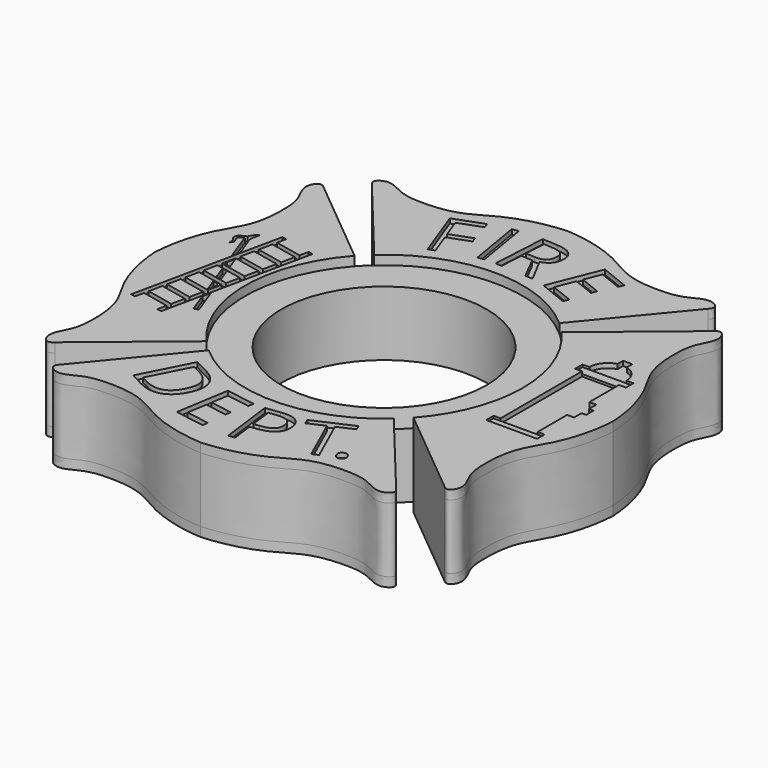
from build123d import *

# Parameters (mm, degrees)
F0_R            = 11.1
F1_DEPTH        = 7
F2_DEPTH        = 8
F3_DEPTH        = 1
F5_DEPTH        = 9.5
F6_DEPTH        = 0.5
F7_DEPTH        = 1
F9_DEPTH        = 9.5
F10_DEPTH       = 0.25
F11_DEPTH       = 0.5
F13_DEPTH       = 0.75
F14_DEPTH       = 1
F15_TEXT_SIZE   = 8.3333333333
F15_TEXT_SIZE_2 = 8.3471097203
F16_DEPTH       = 0.5
F17_TEXT_SIZE   = 8.3333333333
F17_TEXT_SIZE_2 = 8.125
F18_DEPTH       = 0.5


# Not quite as in the source:
# - Text() gives the source's letters only with a copy of the font that has no kerning and outlines rounded to 1/6400 em; it was checked with that copy


with BuildPart() as f1:
    # F0 (on Top) → F1 (new body)
    with BuildSketch(Plane.XY):
        with BuildLine():
            ThreePointArc((-11.1803398875, -10), (-15, 0), (-11.1803398875, 10))
            Line((-11.1803398875, 10), (-21.0544988513, 18.1538552022))
            add(Edge.make_bspline(
                [(-21.0544988513, 18.1538552022), (-21.4950011151, 18.5812700665), (-22.1300751643, 18.2333823026), (-22.4613402272, 16.9307561885), (-21.2849791288, 15.2167799257), (-21.0671926921, 12.725478547), (-21.3396788346, 9.0490697928), (-23.5217250696, 6.0536176188), (-24.5760919224, 2.2657519289), (-24.7081988852, 0.6627934752), (-24.7611551091, 0)],
                knots=[0, 0, 0, 0, 0.0790627116, 0.1662291191, 0.279613322, 0.4082260353, 0.5616601797, 0.7190317703, 0.8790842796, 1, 1, 1, 1], degree=3))
            add(Edge.make_bspline(
                [(-21.0544988513, -18.1538552022), (-21.4950011151, -18.5812700665), (-22.1300751643, -18.2333823026), (-22.4613402272, -16.9307561885), (-21.2849791288, -15.2167799257), (-21.0671926921, -12.725478547), (-21.3396788346, -9.0490697928), (-23.5217250696, -6.0536176188), (-24.5760919224, -2.2657519289), (-24.7081988852, -0.6627934752), (-24.7611551091, 0)],
                knots=[0, 0, 0, 0, 0.0790627116, 0.1662291191, 0.279613322, 0.4082260353, 0.5616601797, 0.7190317703, 0.8790842796, 1, 1, 1, 1], degree=3))
            Line((-21.0544988513, -18.1538552022), (-11.1803398875, -10))
        make_face()
        with BuildLine():
            ThreePointArc((-10, 11.1803398875), (0, 15), (10, 11.1803398875))
            Line((10, 11.1803398875), (18.1538552022, 21.0544988513))
            add(Edge.make_bspline(
                [(18.1538552022, 21.0544988513), (18.5812700665, 21.4950011151), (18.2333823026, 22.1300751643), (16.9307561885, 22.4613402272), (15.2167799257, 21.2849791288), (12.725478547, 21.0671926921), (9.0490697928, 21.3396788346), (6.0536176188, 23.5217250696), (2.2657519289, 24.5760919224), (0.6627934752, 24.7081988852), (0, 24.7611551091)],
                knots=[0, 0, 0, 0, 0.0790627116, 0.1662291191, 0.279613322, 0.4082260353, 0.5616601797, 0.7190317703, 0.8790842796, 1, 1, 1, 1], degree=3))
            add(Edge.make_bspline(
                [(-18.1538552022, 21.0544988513), (-18.5812700665, 21.4950011151), (-18.2333823026, 22.1300751643), (-16.9307561885, 22.4613402272), (-15.2167799257, 21.2849791288), (-12.725478547, 21.0671926921), (-9.0490697928, 21.3396788346), (-6.0536176188, 23.5217250696), (-2.2657519289, 24.5760919224), (-0.6627934752, 24.7081988852), (0, 24.7611551091)],
                knots=[0, 0, 0, 0, 0.0790627116, 0.1662291191, 0.279613322, 0.4082260353, 0.5616601797, 0.7190317703, 0.8790842796, 1, 1, 1, 1], degree=3))
            Line((-18.1538552022, 21.0544988513), (-10, 11.1803398875))
        make_face()
        with BuildLine():
            ThreePointArc((11.1803398875, 10), (14.0125853844, 5.3523313466), (15, 0))
            ThreePointArc((15, 0), (14.0125853844, -5.3523313466), (11.1803398875, -10))
            Line((11.1803398875, -10), (21.0544988513, -18.1538552022))
            add(Edge.make_bspline(
                [(21.0544988513, -18.1538552022), (21.4950011151, -18.5812700665), (22.1300751643, -18.2333823026), (22.4613402272, -16.9307561885), (21.2849791288, -15.2167799257), (21.0671926921, -12.725478547), (21.3396788346, -9.0490697928), (23.5217250696, -6.0536176188), (24.5760919224, -2.2657519289), (24.7081988852, -0.6627934752), (24.7611551091, 0)],
                knots=[0, 0, 0, 0, 0.0790627116, 0.1662291191, 0.279613322, 0.4082260353, 0.5616601797, 0.7190317703, 0.8790842796, 1, 1, 1, 1], degree=3))
            add(Edge.make_bspline(
                [(21.0544988513, 18.1538552022), (21.4950011151, 18.5812700665), (22.1300751643, 18.2333823026), (22.4613402272, 16.9307561885), (21.2849791288, 15.2167799257), (21.0671926921, 12.725478547), (21.3396788346, 9.0490697928), (23.5217250696, 6.0536176188), (24.5760919224, 2.2657519289), (24.7081988852, 0.6627934752), (24.7611551091, 0)],
                knots=[0, 0, 0, 0, 0.0790627116, 0.1662291191, 0.279613322, 0.4082260353, 0.5616601797, 0.7190317703, 0.8790842796, 1, 1, 1, 1], degree=3))
            Line((21.0544988513, 18.1538552022), (11.1803398875, 10))
        make_face()
        with BuildLine():
            Line((18.1538552022, -21.0544988513), (10, -11.1803398875))
            ThreePointArc((10, -11.1803398875), (0, -15), (-10, -11.1803398875))
            Line((-10, -11.1803398875), (-18.1538552022, -21.0544988513))
            add(Edge.make_bspline(
                [(-18.1538552022, -21.0544988513), (-18.5812700665, -21.4950011151), (-18.2333823026, -22.1300751643), (-16.9307561885, -22.4613402272), (-15.2167799257, -21.2849791288), (-12.725478547, -21.0671926921), (-9.0490697928, -21.3396788346), (-6.0536176188, -23.5217250696), (-2.2657519289, -24.5760919224), (-0.6627934752, -24.7081988852), (0, -24.7611551091)],
                knots=[0, 0, 0, 0, 0.0790627116, 0.1662291191, 0.279613322, 0.4082260353, 0.5616601797, 0.7190317703, 0.8790842796, 1, 1, 1, 1], degree=3))
            add(Edge.make_bspline(
                [(18.1538552022, -21.0544988513), (18.5812700665, -21.4950011151), (18.2333823026, -22.1300751643), (16.9307561885, -22.4613402272), (15.2167799257, -21.2849791288), (12.725478547, -21.0671926921), (9.0490697928, -21.3396788346), (6.0536176188, -23.5217250696), (2.2657519289, -24.5760919224), (0.6627934752, -24.7081988852), (0, -24.7611551091)],
                knots=[0, 0, 0, 0, 0.0790627116, 0.1662291191, 0.279613322, 0.4082260353, 0.5616601797, 0.7190317703, 0.8790842796, 1, 1, 1, 1], degree=3))
        make_face()
        with BuildLine():
            ThreePointArc((11.1803398875, -10), (14.0125853844, -5.3523313466), (15, 0))
            ThreePointArc((15, 0), (14.0125853844, 5.3523313466), (11.1803398875, 10))
            ThreePointArc((11.1803398875, 10), (10.6066017178, 10.6066017178), (10, 11.1803398875))
            ThreePointArc((10, 11.1803398875), (0, 15), (-10, 11.1803398875))
            ThreePointArc((-10, 11.1803398875), (-10.6066017178, 10.6066017178), (-11.1803398875, 10))
            ThreePointArc((-11.1803398875, 10), (-15, 0), (-11.1803398875, -10))
            ThreePointArc((-11.1803398875, -10), (-10.6066017178, -10.6066017178), (-10, -11.1803398875))
            ThreePointArc((-10, -11.1803398875), (0, -15), (10, -11.1803398875))
            ThreePointArc((10, -11.1803398875), (10.6066017178, -10.6066017178), (11.1803398875, -10))
        make_face()
        Circle(F0_R, mode=Mode.SUBTRACT)
    extrude(amount=F1_DEPTH)

    # F0 (on Top) → F2 (join)
    with BuildSketch(Plane.XY):
        with BuildLine():
            ThreePointArc((-10, 11.1803398875), (0, 15), (10, 11.1803398875))
            Line((10, 11.1803398875), (18.1538552022, 21.0544988513))
            add(Edge.make_bspline(
                [(18.1538552022, 21.0544988513), (18.5812700665, 21.4950011151), (18.2333823026, 22.1300751643), (16.9307561885, 22.4613402272), (15.2167799257, 21.2849791288), (12.725478547, 21.0671926921), (9.0490697928, 21.3396788346), (6.0536176188, 23.5217250696), (2.2657519289, 24.5760919224), (0.6627934752, 24.7081988852), (0, 24.7611551091)],
                knots=[0, 0, 0, 0, 0.0790627116, 0.1662291191, 0.279613322, 0.4082260353, 0.5616601797, 0.7190317703, 0.8790842796, 1, 1, 1, 1], degree=3))
            add(Edge.make_bspline(
                [(-18.1538552022, 21.0544988513), (-18.5812700665, 21.4950011151), (-18.2333823026, 22.1300751643), (-16.9307561885, 22.4613402272), (-15.2167799257, 21.2849791288), (-12.725478547, 21.0671926921), (-9.0490697928, 21.3396788346), (-6.0536176188, 23.5217250696), (-2.2657519289, 24.5760919224), (-0.6627934752, 24.7081988852), (0, 24.7611551091)],
                knots=[0, 0, 0, 0, 0.0790627116, 0.1662291191, 0.279613322, 0.4082260353, 0.5616601797, 0.7190317703, 0.8790842796, 1, 1, 1, 1], degree=3))
            Line((-18.1538552022, 21.0544988513), (-10, 11.1803398875))
        make_face()
        with BuildLine():
            ThreePointArc((-11.1803398875, -10), (-15, 0), (-11.1803398875, 10))
            Line((-11.1803398875, 10), (-21.0544988513, 18.1538552022))
            add(Edge.make_bspline(
                [(-21.0544988513, 18.1538552022), (-21.4950011151, 18.5812700665), (-22.1300751643, 18.2333823026), (-22.4613402272, 16.9307561885), (-21.2849791288, 15.2167799257), (-21.0671926921, 12.725478547), (-21.3396788346, 9.0490697928), (-23.5217250696, 6.0536176188), (-24.5760919224, 2.2657519289), (-24.7081988852, 0.6627934752), (-24.7611551091, 0)],
                knots=[0, 0, 0, 0, 0.0790627116, 0.1662291191, 0.279613322, 0.4082260353, 0.5616601797, 0.7190317703, 0.8790842796, 1, 1, 1, 1], degree=3))
            add(Edge.make_bspline(
                [(-21.0544988513, -18.1538552022), (-21.4950011151, -18.5812700665), (-22.1300751643, -18.2333823026), (-22.4613402272, -16.9307561885), (-21.2849791288, -15.2167799257), (-21.0671926921, -12.725478547), (-21.3396788346, -9.0490697928), (-23.5217250696, -6.0536176188), (-24.5760919224, -2.2657519289), (-24.7081988852, -0.6627934752), (-24.7611551091, 0)],
                knots=[0, 0, 0, 0, 0.0790627116, 0.1662291191, 0.279613322, 0.4082260353, 0.5616601797, 0.7190317703, 0.8790842796, 1, 1, 1, 1], degree=3))
            Line((-21.0544988513, -18.1538552022), (-11.1803398875, -10))
        make_face()
        with BuildLine():
            Line((18.1538552022, -21.0544988513), (10, -11.1803398875))
            ThreePointArc((10, -11.1803398875), (0, -15), (-10, -11.1803398875))
            Line((-10, -11.1803398875), (-18.1538552022, -21.0544988513))
            add(Edge.make_bspline(
                [(-18.1538552022, -21.0544988513), (-18.5812700665, -21.4950011151), (-18.2333823026, -22.1300751643), (-16.9307561885, -22.4613402272), (-15.2167799257, -21.2849791288), (-12.725478547, -21.0671926921), (-9.0490697928, -21.3396788346), (-6.0536176188, -23.5217250696), (-2.2657519289, -24.5760919224), (-0.6627934752, -24.7081988852), (0, -24.7611551091)],
                knots=[0, 0, 0, 0, 0.0790627116, 0.1662291191, 0.279613322, 0.4082260353, 0.5616601797, 0.7190317703, 0.8790842796, 1, 1, 1, 1], degree=3))
            add(Edge.make_bspline(
                [(18.1538552022, -21.0544988513), (18.5812700665, -21.4950011151), (18.2333823026, -22.1300751643), (16.9307561885, -22.4613402272), (15.2167799257, -21.2849791288), (12.725478547, -21.0671926921), (9.0490697928, -21.3396788346), (6.0536176188, -23.5217250696), (2.2657519289, -24.5760919224), (0.6627934752, -24.7081988852), (0, -24.7611551091)],
                knots=[0, 0, 0, 0, 0.0790627116, 0.1662291191, 0.279613322, 0.4082260353, 0.5616601797, 0.7190317703, 0.8790842796, 1, 1, 1, 1], degree=3))
        make_face()
        with BuildLine():
            ThreePointArc((11.1803398875, 10), (14.0125853844, 5.3523313466), (15, 0))
            ThreePointArc((15, 0), (14.0125853844, -5.3523313466), (11.1803398875, -10))
            Line((11.1803398875, -10), (21.0544988513, -18.1538552022))
            add(Edge.make_bspline(
                [(21.0544988513, -18.1538552022), (21.4950011151, -18.5812700665), (22.1300751643, -18.2333823026), (22.4613402272, -16.9307561885), (21.2849791288, -15.2167799257), (21.0671926921, -12.725478547), (21.3396788346, -9.0490697928), (23.5217250696, -6.0536176188), (24.5760919224, -2.2657519289), (24.7081988852, -0.6627934752), (24.7611551091, 0)],
                knots=[0, 0, 0, 0, 0.0790627116, 0.1662291191, 0.279613322, 0.4082260353, 0.5616601797, 0.7190317703, 0.8790842796, 1, 1, 1, 1], degree=3))
            add(Edge.make_bspline(
                [(21.0544988513, 18.1538552022), (21.4950011151, 18.5812700665), (22.1300751643, 18.2333823026), (22.4613402272, 16.9307561885), (21.2849791288, 15.2167799257), (21.0671926921, 12.725478547), (21.3396788346, 9.0490697928), (23.5217250696, 6.0536176188), (24.5760919224, 2.2657519289), (24.7081988852, 0.6627934752), (24.7611551091, 0)],
                knots=[0, 0, 0, 0, 0.0790627116, 0.1662291191, 0.279613322, 0.4082260353, 0.5616601797, 0.7190317703, 0.8790842796, 1, 1, 1, 1], degree=3))
            Line((21.0544988513, 18.1538552022), (11.1803398875, 10))
        make_face()
    extrude(amount=F2_DEPTH)

    # F0 (on Top) → F3 (join)
    with BuildSketch(Plane.XY):
        with BuildLine():
            ThreePointArc((-10, 11.1803398875), (0, 15), (10, 11.1803398875))
            Line((10, 11.1803398875), (18.1538552022, 21.0544988513))
            add(Edge.make_bspline(
                [(18.1538552022, 21.0544988513), (18.5812700665, 21.4950011151), (18.2333823026, 22.1300751643), (16.9307561885, 22.4613402272), (15.2167799257, 21.2849791288), (12.725478547, 21.0671926921), (9.0490697928, 21.3396788346), (6.0536176188, 23.5217250696), (2.2657519289, 24.5760919224), (0.6627934752, 24.7081988852), (0, 24.7611551091)],
                knots=[0, 0, 0, 0, 0.0790627116, 0.1662291191, 0.279613322, 0.4082260353, 0.5616601797, 0.7190317703, 0.8790842796, 1, 1, 1, 1], degree=3))
            add(Edge.make_bspline(
                [(-18.1538552022, 21.0544988513), (-18.5812700665, 21.4950011151), (-18.2333823026, 22.1300751643), (-16.9307561885, 22.4613402272), (-15.2167799257, 21.2849791288), (-12.725478547, 21.0671926921), (-9.0490697928, 21.3396788346), (-6.0536176188, 23.5217250696), (-2.2657519289, 24.5760919224), (-0.6627934752, 24.7081988852), (0, 24.7611551091)],
                knots=[0, 0, 0, 0, 0.0790627116, 0.1662291191, 0.279613322, 0.4082260353, 0.5616601797, 0.7190317703, 0.8790842796, 1, 1, 1, 1], degree=3))
            Line((-18.1538552022, 21.0544988513), (-10, 11.1803398875))
        make_face()
        with BuildLine():
            ThreePointArc((-11.1803398875, -10), (-15, 0), (-11.1803398875, 10))
            Line((-11.1803398875, 10), (-21.0544988513, 18.1538552022))
            add(Edge.make_bspline(
                [(-21.0544988513, 18.1538552022), (-21.4950011151, 18.5812700665), (-22.1300751643, 18.2333823026), (-22.4613402272, 16.9307561885), (-21.2849791288, 15.2167799257), (-21.0671926921, 12.725478547), (-21.3396788346, 9.0490697928), (-23.5217250696, 6.0536176188), (-24.5760919224, 2.2657519289), (-24.7081988852, 0.6627934752), (-24.7611551091, 0)],
                knots=[0, 0, 0, 0, 0.0790627116, 0.1662291191, 0.279613322, 0.4082260353, 0.5616601797, 0.7190317703, 0.8790842796, 1, 1, 1, 1], degree=3))
            add(Edge.make_bspline(
                [(-21.0544988513, -18.1538552022), (-21.4950011151, -18.5812700665), (-22.1300751643, -18.2333823026), (-22.4613402272, -16.9307561885), (-21.2849791288, -15.2167799257), (-21.0671926921, -12.725478547), (-21.3396788346, -9.0490697928), (-23.5217250696, -6.0536176188), (-24.5760919224, -2.2657519289), (-24.7081988852, -0.6627934752), (-24.7611551091, 0)],
                knots=[0, 0, 0, 0, 0.0790627116, 0.1662291191, 0.279613322, 0.4082260353, 0.5616601797, 0.7190317703, 0.8790842796, 1, 1, 1, 1], degree=3))
            Line((-21.0544988513, -18.1538552022), (-11.1803398875, -10))
        make_face()
        with BuildLine():
            Line((18.1538552022, -21.0544988513), (10, -11.1803398875))
            ThreePointArc((10, -11.1803398875), (0, -15), (-10, -11.1803398875))
            Line((-10, -11.1803398875), (-18.1538552022, -21.0544988513))
            add(Edge.make_bspline(
                [(-18.1538552022, -21.0544988513), (-18.5812700665, -21.4950011151), (-18.2333823026, -22.1300751643), (-16.9307561885, -22.4613402272), (-15.2167799257, -21.2849791288), (-12.725478547, -21.0671926921), (-9.0490697928, -21.3396788346), (-6.0536176188, -23.5217250696), (-2.2657519289, -24.5760919224), (-0.6627934752, -24.7081988852), (0, -24.7611551091)],
                knots=[0, 0, 0, 0, 0.0790627116, 0.1662291191, 0.279613322, 0.4082260353, 0.5616601797, 0.7190317703, 0.8790842796, 1, 1, 1, 1], degree=3))
            add(Edge.make_bspline(
                [(18.1538552022, -21.0544988513), (18.5812700665, -21.4950011151), (18.2333823026, -22.1300751643), (16.9307561885, -22.4613402272), (15.2167799257, -21.2849791288), (12.725478547, -21.0671926921), (9.0490697928, -21.3396788346), (6.0536176188, -23.5217250696), (2.2657519289, -24.5760919224), (0.6627934752, -24.7081988852), (0, -24.7611551091)],
                knots=[0, 0, 0, 0, 0.0790627116, 0.1662291191, 0.279613322, 0.4082260353, 0.5616601797, 0.7190317703, 0.8790842796, 1, 1, 1, 1], degree=3))
        make_face()
        with BuildLine():
            ThreePointArc((11.1803398875, 10), (14.0125853844, 5.3523313466), (15, 0))
            ThreePointArc((15, 0), (14.0125853844, -5.3523313466), (11.1803398875, -10))
            Line((11.1803398875, -10), (21.0544988513, -18.1538552022))
            add(Edge.make_bspline(
                [(21.0544988513, -18.1538552022), (21.4950011151, -18.5812700665), (22.1300751643, -18.2333823026), (22.4613402272, -16.9307561885), (21.2849791288, -15.2167799257), (21.0671926921, -12.725478547), (21.3396788346, -9.0490697928), (23.5217250696, -6.0536176188), (24.5760919224, -2.2657519289), (24.7081988852, -0.6627934752), (24.7611551091, 0)],
                knots=[0, 0, 0, 0, 0.0790627116, 0.1662291191, 0.279613322, 0.4082260353, 0.5616601797, 0.7190317703, 0.8790842796, 1, 1, 1, 1], degree=3))
            add(Edge.make_bspline(
                [(21.0544988513, 18.1538552022), (21.4950011151, 18.5812700665), (22.1300751643, 18.2333823026), (22.4613402272, 16.9307561885), (21.2849791288, 15.2167799257), (21.0671926921, 12.725478547), (21.3396788346, 9.0490697928), (23.5217250696, 6.0536176188), (24.5760919224, 2.2657519289), (24.7081988852, 0.6627934752), (24.7611551091, 0)],
                knots=[0, 0, 0, 0, 0.0790627116, 0.1662291191, 0.279613322, 0.4082260353, 0.5616601797, 0.7190317703, 0.8790842796, 1, 1, 1, 1], degree=3))
            Line((21.0544988513, 18.1538552022), (11.1803398875, 10))
        make_face()
    extrude(amount=-F3_DEPTH)

    # F4 (on face) → F5 (join)
    with BuildSketch(Plane.XY.offset(8)):
        with BuildLine():
            Line((-19.2767570017, 3.5073122645), (-19.081227367, 4.4241287993))
            Line((-19.081227367, 4.4241287993), (-19.7800920275, 6.3241662521))
            add(Edge.make_bspline(
                [(-19.7800920275, 6.3241662521), (-19.8797484646, 6.5374998472), (-20.0881030853, 6.983522619), (-19.7129121529, 7.8695591923), (-19.8691599668, 8.0166589982), (-20.2628380693, 7.5138888966), (-20.4072439128, 7.2370915766), (-20.4347793507, 7.1311267456)],
                knots=[0, 0, 0, 0, 0.1889010167, 0.3949408674, 0.4592615309, 0.6375996822, 0.741788244, 0.741788244, 0.741788244, 0.741788244], degree=3))
            add(Edge.make_bspline(
                [(-20.4347793507, 7.1311267456), (-20.450259938, 7.0715526862), (-20.4634094461, 6.9627999345), (-20.4495616456, 6.8376419519), (-20.4394222839, 6.7800081977)],
                knots=[0.741788244, 0.741788244, 0.741788244, 0.741788244, 0.8003636743, 0.8465562021, 0.8465562021, 0.8465562021, 0.8465562021], degree=3))
            add(Edge.make_bspline(
                [(-20.4394222839, 6.7800081977), (-20.4057410323, 6.588558573), (-20.3275483083, 6.3700610305), (-20.2493555844, 6.1515634879)],
                knots=[0.8465562021, 0.8465562021, 0.8465562021, 0.8465562021, 1, 1, 1, 1], degree=3))
            Line((-20.2493555844, 6.1515634879), (-19.2767570017, 3.5073122645))
        make_face()
        with BuildLine():
            add(Edge.make_bspline(
                [(-20.4347793507, 7.1311267456), (-20.450259938, 7.0715526862), (-20.4634094461, 6.9627999345), (-20.4495616456, 6.8376419519), (-20.4394222839, 6.7800081977)],
                knots=[0.741788244, 0.741788244, 0.741788244, 0.741788244, 0.8003636743, 0.8465562021, 0.8465562021, 0.8465562021, 0.8465562021], degree=3))
            add(Edge.make_bspline(
                [(-20.4347793507, 7.1311267456), (-20.6981350566, 7.0123843934), (-21.1252316698, 6.8193710677), (-21.2735510779, 6.5345468024), (-21.3330718318, 6.2409512841), (-21.1029653015, 5.9941350375), (-20.8947353864, 5.6348757789), (-20.9523179302, 5.4115023528), (-20.9796205163, 5.3055896424)],
                knots=[0, 0, 0, 0, 0.2359057691, 0.3829791313, 0.5212865528, 0.6750607493, 0.8459442462, 1, 1, 1, 1], degree=3))
            add(Edge.make_bspline(
                [(-20.4394222839, 6.7800081977), (-20.5997238295, 6.7086329249), (-20.8490962685, 6.5973842442), (-20.9332462706, 6.4617054533), (-20.9570883394, 6.3103192594), (-20.91062343, 6.0931301517), (-20.6526137697, 5.6439462742), (-20.8720837955, 5.4168590409), (-20.9796205163, 5.3055896424)],
                knots=[0, 0, 0, 0, 0.2091684458, 0.3259978825, 0.4408852214, 0.5880681011, 0.7982024917, 1, 1, 1, 1], degree=3))
        make_face()
        Polygon((-17.8920581902, 7.2938867548), (-17.7877684886, 7.7828894728), (-17.5791890855, 8.7608949087), (-18.0681918034, 8.8651846102), (-21.5097519552, -7.2719050816), (-21.0207492373, -7.3761947832), (-20.8121698341, -6.3981893473), (-20.7078801326, -5.9091866294), (-20.3950110279, -4.4421784756), (-20.2907213263, -3.9531757576), (-19.9778522216, -2.4861676038), (-19.87356252, -1.9971648859), (-19.5606934153, -0.5301567321), (-19.4564037137, -0.0411540142), (-19.143534609, 1.4258541396), (-19.0392449074, 1.9148568576), (-18.7263758027, 3.3818650114), (-18.6220861012, 3.8708677293), (-18.3092169965, 5.3378758831), (-18.2049272949, 5.826878601), align=None)
        Polygon((-17.5977302117, -8.1062226941), (-14.1561700599, 8.0308669977), (-14.6451727779, 8.1351566992), (-14.853752181, 7.1571512634), (-14.9580418826, 6.6681485454), (-15.2709109873, 5.2011403916), (-15.3752006888, 4.7121376737), (-15.6880697936, 3.2451295199), (-15.7923594951, 2.756126802), (-16.1052285998, 1.2891186482), (-16.2095183014, 0.8001159302), (-16.5223874061, -0.6668922236), (-16.6266771077, -1.1558949415), (-16.9395462124, -2.6229030953), (-17.043835914, -3.1119058132), (-17.3567050187, -4.578913967), (-17.4609947203, -5.067916685), (-17.773863825, -6.5349248388), (-17.8781535265, -7.0239275567), (-18.0867329297, -8.0019329926), align=None)
        Polygon((-14.9580418826, 6.6681485454), (-14.853752181, 7.1571512634), (-17.7877684886, 7.7828894728), (-17.8920581902, 7.2938867548), align=None)
        Polygon((-15.3752006888, 4.7121376737), (-15.2709109873, 5.2011403916), (-18.2049272949, 5.826878601), (-18.3092169965, 5.3378758831), align=None)
        Polygon((-15.7923594951, 2.756126802), (-15.6880697936, 3.2451295199), (-18.6220861012, 3.8708677293), (-18.7263758027, 3.3818650114), align=None)
        Polygon((-18.8739320775, 2.4121324874), (-18.6946000196, 1.9245736713), (-18.1219706332, 1.8161507112), (-18.6784024427, 3.3289490223), align=None)
        Polygon((-16.2095183014, 0.8001159302), (-16.1052285998, 1.2891186482), (-19.0392449074, 1.9148568576), (-19.143534609, 1.4258541396), align=None)
        Polygon((-17.8491255484, 1.0743534661), (-18.4272236771, 1.1976445627), (-17.881912486, -0.2849195805), (-17.3038143573, -0.4082106771), align=None)
        Polygon((-19.5606934153, -0.5301567321), (-16.6266771077, -1.1558949415), (-16.5223874061, -0.6668922236), (-19.4564037137, -0.0411540142), align=None)
        Polygon((-17.0168768688, -1.188321628), (-17.5949749974, -1.0650305314), (-17.0796403416, -2.4660960052), (-17.0156201146, -2.479749611), (-16.8417439864, -1.6644639406), align=None)
        Polygon((-19.9778522216, -2.4861676038), (-17.043835914, -3.1119058132), (-16.9395462124, -2.6229030953), (-19.87356252, -1.9971648859), align=None)
        Polygon((-20.3950110279, -4.4421784756), (-17.4609947203, -5.067916685), (-17.3567050187, -4.578913967), (-20.2907213263, -3.9531757576), align=None)
        Polygon((-20.8121698341, -6.3981893473), (-17.8781535265, -7.0239275567), (-17.773863825, -6.5349248388), (-20.7078801326, -5.9091866294), align=None)
        Polygon((-16.5816127725, -3.8201078582), (-15.7611500472, -6.050739903), (-15.2918864903, -5.8781371388), (-16.3860831378, -2.9032913234), align=None)
    extrude(amount=-F5_DEPTH)

    # F4 (on face) → F6 (cut)
    with BuildSketch(Plane.XY.offset(8)):
        with BuildLine():
            Line((-19.2767570017, 3.5073122645), (-19.081227367, 4.4241287993))
            Line((-19.081227367, 4.4241287993), (-19.7800920275, 6.3241662521))
            add(Edge.make_bspline(
                [(-19.7800920275, 6.3241662521), (-19.8797484646, 6.5374998472), (-20.0881030853, 6.983522619), (-19.7129121529, 7.8695591923), (-19.8691599668, 8.0166589982), (-20.2628380693, 7.5138888966), (-20.4072439128, 7.2370915766), (-20.4347793507, 7.1311267456)],
                knots=[0, 0, 0, 0, 0.1889010167, 0.3949408674, 0.4592615309, 0.6375996822, 0.741788244, 0.741788244, 0.741788244, 0.741788244], degree=3))
            add(Edge.make_bspline(
                [(-20.4347793507, 7.1311267456), (-20.450259938, 7.0715526862), (-20.4634094461, 6.9627999345), (-20.4495616456, 6.8376419519), (-20.4394222839, 6.7800081977)],
                knots=[0.741788244, 0.741788244, 0.741788244, 0.741788244, 0.8003636743, 0.8465562021, 0.8465562021, 0.8465562021, 0.8465562021], degree=3))
            add(Edge.make_bspline(
                [(-20.4394222839, 6.7800081977), (-20.4057410323, 6.588558573), (-20.3275483083, 6.3700610305), (-20.2493555844, 6.1515634879)],
                knots=[0.8465562021, 0.8465562021, 0.8465562021, 0.8465562021, 1, 1, 1, 1], degree=3))
            Line((-20.2493555844, 6.1515634879), (-19.2767570017, 3.5073122645))
        make_face()
        with BuildLine():
            add(Edge.make_bspline(
                [(-20.4347793507, 7.1311267456), (-20.450259938, 7.0715526862), (-20.4634094461, 6.9627999345), (-20.4495616456, 6.8376419519), (-20.4394222839, 6.7800081977)],
                knots=[0.741788244, 0.741788244, 0.741788244, 0.741788244, 0.8003636743, 0.8465562021, 0.8465562021, 0.8465562021, 0.8465562021], degree=3))
            add(Edge.make_bspline(
                [(-20.4347793507, 7.1311267456), (-20.6981350566, 7.0123843934), (-21.1252316698, 6.8193710677), (-21.2735510779, 6.5345468024), (-21.3330718318, 6.2409512841), (-21.1029653015, 5.9941350375), (-20.8947353864, 5.6348757789), (-20.9523179302, 5.4115023528), (-20.9796205163, 5.3055896424)],
                knots=[0, 0, 0, 0, 0.2359057691, 0.3829791313, 0.5212865528, 0.6750607493, 0.8459442462, 1, 1, 1, 1], degree=3))
            add(Edge.make_bspline(
                [(-20.4394222839, 6.7800081977), (-20.5997238295, 6.7086329249), (-20.8490962685, 6.5973842442), (-20.9332462706, 6.4617054533), (-20.9570883394, 6.3103192594), (-20.91062343, 6.0931301517), (-20.6526137697, 5.6439462742), (-20.8720837955, 5.4168590409), (-20.9796205163, 5.3055896424)],
                knots=[0, 0, 0, 0, 0.2091684458, 0.3259978825, 0.4408852214, 0.5880681011, 0.7982024917, 1, 1, 1, 1], degree=3))
        make_face()
        Polygon((-17.8920581902, 7.2938867548), (-17.7877684886, 7.7828894728), (-17.5791890855, 8.7608949087), (-18.0681918034, 8.8651846102), (-21.5097519552, -7.2719050816), (-21.0207492373, -7.3761947832), (-20.8121698341, -6.3981893473), (-20.7078801326, -5.9091866294), (-20.3950110279, -4.4421784756), (-20.2907213263, -3.9531757576), (-19.9778522216, -2.4861676038), (-19.87356252, -1.9971648859), (-19.5606934153, -0.5301567321), (-19.4564037137, -0.0411540142), (-19.143534609, 1.4258541396), (-19.0392449074, 1.9148568576), (-18.7263758027, 3.3818650114), (-18.6220861012, 3.8708677293), (-18.3092169965, 5.3378758831), (-18.2049272949, 5.826878601), align=None)
        Polygon((-14.9580418826, 6.6681485454), (-14.853752181, 7.1571512634), (-17.7877684886, 7.7828894728), (-17.8920581902, 7.2938867548), align=None)
        Polygon((-17.5977302117, -8.1062226941), (-14.1561700599, 8.0308669977), (-14.6451727779, 8.1351566992), (-14.853752181, 7.1571512634), (-14.9580418826, 6.6681485454), (-15.2709109873, 5.2011403916), (-15.3752006888, 4.7121376737), (-15.6880697936, 3.2451295199), (-15.7923594951, 2.756126802), (-16.1052285998, 1.2891186482), (-16.2095183014, 0.8001159302), (-16.5223874061, -0.6668922236), (-16.6266771077, -1.1558949415), (-16.9395462124, -2.6229030953), (-17.043835914, -3.1119058132), (-17.3567050187, -4.578913967), (-17.4609947203, -5.067916685), (-17.773863825, -6.5349248388), (-17.8781535265, -7.0239275567), (-18.0867329297, -8.0019329926), align=None)
        Polygon((-15.3752006888, 4.7121376737), (-15.2709109873, 5.2011403916), (-18.2049272949, 5.826878601), (-18.3092169965, 5.3378758831), align=None)
        Polygon((-15.7923594951, 2.756126802), (-15.6880697936, 3.2451295199), (-18.6220861012, 3.8708677293), (-18.7263758027, 3.3818650114), align=None)
        Polygon((-18.8739320775, 2.4121324874), (-18.6946000196, 1.9245736713), (-18.1219706332, 1.8161507112), (-18.6784024427, 3.3289490223), align=None)
        Polygon((-16.2095183014, 0.8001159302), (-16.1052285998, 1.2891186482), (-19.0392449074, 1.9148568576), (-19.143534609, 1.4258541396), align=None)
        Polygon((-17.8491255484, 1.0743534661), (-18.4272236771, 1.1976445627), (-17.881912486, -0.2849195805), (-17.3038143573, -0.4082106771), align=None)
        Polygon((-19.5606934153, -0.5301567321), (-16.6266771077, -1.1558949415), (-16.5223874061, -0.6668922236), (-19.4564037137, -0.0411540142), align=None)
        Polygon((-17.0168768688, -1.188321628), (-17.5949749974, -1.0650305314), (-17.0796403416, -2.4660960052), (-17.0156201146, -2.479749611), (-16.8417439864, -1.6644639406), align=None)
        Polygon((-19.9778522216, -2.4861676038), (-17.043835914, -3.1119058132), (-16.9395462124, -2.6229030953), (-19.87356252, -1.9971648859), align=None)
        Polygon((-20.3950110279, -4.4421784756), (-17.4609947203, -5.067916685), (-17.3567050187, -4.578913967), (-20.2907213263, -3.9531757576), align=None)
        Polygon((-20.8121698341, -6.3981893473), (-17.8781535265, -7.0239275567), (-17.773863825, -6.5349248388), (-20.7078801326, -5.9091866294), align=None)
        Polygon((-16.5816127725, -3.8201078582), (-15.7611500472, -6.050739903), (-15.2918864903, -5.8781371388), (-16.3860831378, -2.9032913234), align=None)
    extrude(amount=-F6_DEPTH, mode=Mode.SUBTRACT)

    # F7 (cut): faces of the model
    f7_faces = [f1.faces().sort_by_distance(p)[0] for p in [
        (-21.2266716474, -7.1431575667, -1.5),
        (-20.0435896434, 5.9310692142, -1.5),
        (-18.5594176947, 2.404978517, -1.5),
        (-17.8655190172, 0.3947169428, -1.5),
        (-17.1570956587, -1.6538197449, -1.5),
        (-15.9972627976, -4.6500897664, -1.5),
    ]]
    extrude(f7_faces, amount=-F7_DEPTH, mode=Mode.SUBTRACT)

    # F8 (on face) → F9 (join)
    with BuildSketch(Plane.XY.offset(8)):
        Polygon((21, -5.5), (17, -5.5), (16.25, -5.5), (16.25, -6.5), (21.75, -6.5), (21.75, -5.5), align=None)
        Polygon((17, 5.5), (17, -5.5), (21, -5.5), (21, -1.5), (21, 1.5), (21, 5.5), align=None)
        Polygon((16.25, 5.5), (17, 5.5), (21, 5.5), (21.75, 5.5), (21.75, 6.5), (21, 6.5), (17, 6.5), (16.25, 6.5), align=None)
        Polygon((21, 1.5), (21, -1.5), (21.75, -1.5), (21.75, -0.5), (22.25, -0.5), (22.25, 0.5), (21.75, 0.5), (21.75, 1.5), align=None)
        with BuildLine():
            ThreePointArc((18.5, 8.4257202928), (17.4221534734, 7.7182294187), (17, 6.5))
            Line((17, 6.5), (21, 6.5))
            ThreePointArc((21, 6.5), (20.5778465266, 7.7182294187), (19.5, 8.4257202928))
            ThreePointArc((19.5, 8.4257202928), (19, 8.4892276631), (18.5, 8.4257202928))
        make_face()
        with BuildLine():
            Line((18.5, 9.1757202928), (18.5, 8.4257202928))
            ThreePointArc((18.5, 8.4257202928), (19, 8.4892276631), (19.5, 8.4257202928))
            Line((19.5, 8.4257202928), (19.5, 9.1757202928))
            Line((19.5, 9.1757202928), (18.5, 9.1757202928))
        make_face()
    extrude(amount=-F9_DEPTH)

    # F8 (on face) → F10 (cut)
    with BuildSketch(Plane.XY.offset(8)):
        Polygon((16.25, 5.5), (17, 5.5), (21, 5.5), (21.75, 5.5), (21.75, 6.5), (21, 6.5), (17, 6.5), (16.25, 6.5), align=None)
        Polygon((21, -5.5), (17, -5.5), (16.25, -5.5), (16.25, -6.5), (21.75, -6.5), (21.75, -5.5), align=None)
    extrude(amount=-F10_DEPTH, mode=Mode.SUBTRACT)

    # F8 (on face) → F11 (cut)
    with BuildSketch(Plane.XY.offset(8)):
        Polygon((17, 5.5), (17, -5.5), (21, -5.5), (21, -1.5), (21, 1.5), (21, 5.5), align=None)
        Polygon((21, 1.5), (21, -1.5), (21.75, -1.5), (21.75, -0.5), (22.25, -0.5), (22.25, 0.5), (21.75, 0.5), (21.75, 1.5), align=None)
        with BuildLine():
            ThreePointArc((18.5, 8.4257202928), (17.4221534734, 7.7182294187), (17, 6.5))
            Line((17, 6.5), (21, 6.5))
            ThreePointArc((21, 6.5), (20.5778465266, 7.7182294187), (19.5, 8.4257202928))
            ThreePointArc((19.5, 8.4257202928), (19, 8.4892276631), (18.5, 8.4257202928))
        make_face()
        with BuildLine():
            Line((18.5, 9.1757202928), (18.5, 8.4257202928))
            ThreePointArc((18.5, 8.4257202928), (19, 8.4892276631), (19.5, 8.4257202928))
            Line((19.5, 8.4257202928), (19.5, 9.1757202928))
            Line((19.5, 9.1757202928), (18.5, 9.1757202928))
        make_face()
    extrude(amount=-F11_DEPTH, mode=Mode.SUBTRACT)

    # F12 (on face) → F13 (cut)
    with BuildSketch(Plane(origin=(0, 0, -1.5), x_dir=(1, 0, 0), z_dir=(0, 0, -1))):
        Polygon((17, -6.5), (21, -6.5), (21.75, -6.5), (21.75, -5.5), (21, -5.5), (17, -5.5), (16.25, -5.5), (16.25, -6.5), align=None)
        Polygon((16.25, 5.5), (17, 5.5), (21, 5.5), (21.75, 5.5), (21.75, 6.5), (16.25, 6.5), align=None)
    extrude(amount=-F13_DEPTH, mode=Mode.SUBTRACT)

    # F14 (cut): faces of the model
    f14_faces = [f1.faces().sort_by_distance(p)[0] for p in [
        (19, 7.4943734187, -1.5),
        (19.1463903743, 0, -1.5),
    ]]
    extrude(f14_faces, amount=-F14_DEPTH, mode=Mode.SUBTRACT)

    # F15 (on face) → F16 (cut)
    with BuildSketch(Plane.XY.offset(8)):
        with Locations(Location((-7.8756261506, 14.4991211022), (0, 0, 20.3665177698))):
            Text('F', F15_TEXT_SIZE, font='Open Sans', text_align=(TextAlign.LEFT, TextAlign.BOTTOM))
        with Locations(Location((-3.6959011221, 16.0807436052), (0, 0, 9.383058783))):
            Text('I', F15_TEXT_SIZE, font='Open Sans', text_align=(TextAlign.LEFT, TextAlign.BOTTOM))
        with Locations(Location((-1.8406920479, 16.3970074338), (0, 0, -3.292281681))):
            Text('R', F15_TEXT_SIZE_2, font='Open Sans', text_align=(TextAlign.LEFT, TextAlign.BOTTOM))
        with Locations(Location((3.9125860794, 16.0294001813), (0, 0, -21.8603887627))):
            Text('E', F15_TEXT_SIZE, font='Open Sans', text_align=(TextAlign.LEFT, TextAlign.BOTTOM))
    extrude(amount=-F16_DEPTH, mode=Mode.SUBTRACT)

    # F17 (on face) → F18 (cut)
    with BuildSketch(Plane.XY.offset(8)):
        with Locations(Location((-12.8414565668, -18.3827968461), (0, 0, -27.1104564152))):
            Text('D', F17_TEXT_SIZE, font='Open Sans', text_align=(TextAlign.LEFT, TextAlign.BOTTOM))
        with Locations(Location((-5.845141689, -21.5292083195), (0, 0, -9.3265949988))):
            Text('E', F17_TEXT_SIZE_2, font='Open Sans', text_align=(TextAlign.LEFT, TextAlign.BOTTOM))
        with Locations(Location((0.2122205354, -22.4454380424), (0, 0, 7.1036179248))):
            Text('P', F17_TEXT_SIZE, font='Open Sans', text_align=(TextAlign.LEFT, TextAlign.BOTTOM))
        with Locations(Location((6.8177945305, -21.3872436778), (0, 0, 24.1691265122))):
            Text('T', F17_TEXT_SIZE, font='Open Sans', text_align=(TextAlign.LEFT, TextAlign.BOTTOM))
        with Locations(Location((10.0595431417, -20.1156429141), (0, 0, 29.2949942399))):
            Text('.', F17_TEXT_SIZE, font='Open Sans', text_align=(TextAlign.LEFT, TextAlign.BOTTOM))
    extrude(amount=-F18_DEPTH, mode=Mode.SUBTRACT)


solid = f1.part
